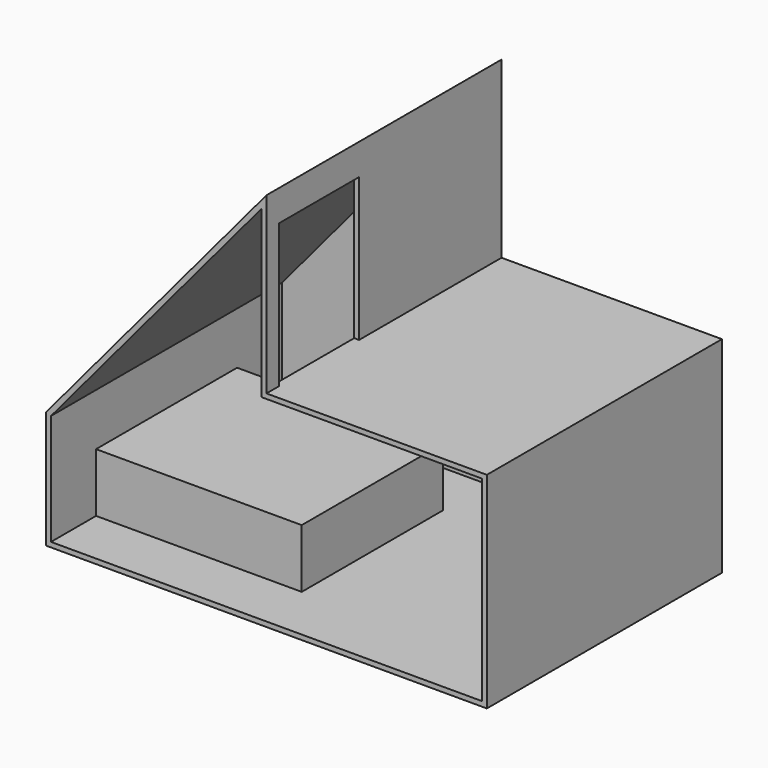
from build123d import *

# Parameters (mm, degrees)
F1_DEPTH = 3000
F2_T     = -50
F3_W     = 1019.7913646698
F3_H     = 1464.2549991608
F4_DEPTH = 50
F5_W     = 2100
F5_H     = 1800
F6_DEPTH = 600
F7_W     = 2000
F7_H     = 1900
F8_DEPTH = 600


with BuildPart() as f1:
    # F0 (on Front) → F1 (new body)
    with BuildSketch(Plane.XZ):
        Polygon((-4401.0416188458, 0), (98.9583811542, 0), (98.9583811542, 2100), (-2151.0416188458, 2100), (-2151.0416188458, 3881.445583337), (-4401.0416188458, 1200), align=None)
    extrude(amount=F1_DEPTH)

    # F2
    f2_openings = [f1.faces().sort_by_distance(p)[0] for p in [
        (-2149.542304, -3000, 1235.201069),
    ]]
    offset(amount=F2_T, openings=f2_openings, kind=Kind.INTERSECTION)

    # F3 (on face) → F4 (cut, through all)
    with BuildSketch(Plane.YZ.offset(-2151.0416188458)):
        with Locations((-2327.8425931931, 2832.1274995804)):
            Rectangle(F3_W, F3_H)
    extrude(amount=-F4_DEPTH, mode=Mode.SUBTRACT)

    # F5 (on face) → F6 (join)
    with BuildSketch(Plane.XY.offset(50)):
        with Locations((-3301.0416188458, -1525)):
            Rectangle(F5_W, F5_H)
    extrude(amount=F6_DEPTH)

    # F7 (on face) → F8 (join)
    with BuildSketch(Plane(origin=(48.9583811542, 0, 0), x_dir=(0, -1, 0), z_dir=(-1, 0, 0))):
        with Locations((1050, 1000)):
            Rectangle(F7_W, F7_H)
    extrude(amount=F8_DEPTH)


solid = f1.part
